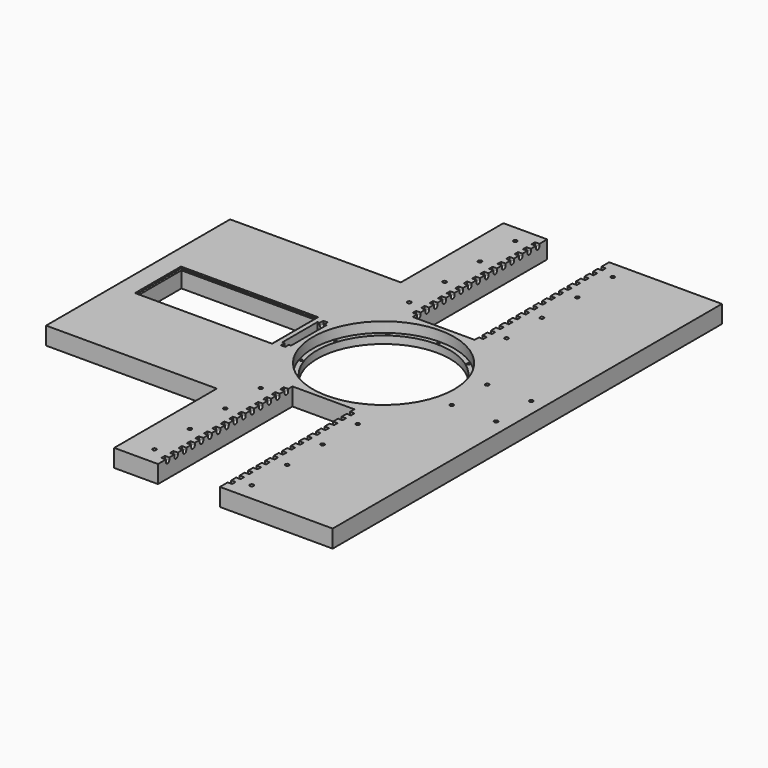
from build123d import *

# Parameters (mm, degrees)
F0_W      = 200
F0_H      = 255
F1_DEPTH  = 20
F2_W      = 150
F2_H      = 60
F3_DEPTH  = 20.001
F4_W      = 155
F4_H      = 65
F4_W_2    = 150
F4_H_2    = 60
F5_DEPTH  = 2
F6_DEPTH  = 240
F7_R      = 75
F8_DEPTH  = 25
F7_R_2    = 80
F9_DEPTH  = 11.5
F10_W     = 170
F10_H     = 147.5
F10_H_2   = 255
F10_R     = 80
F11_DEPTH = 10
F12_W     = 70
F12_H     = 190
F13_DEPTH = 25
F15_W     = 70
F15_H     = 190
F16_DEPTH = 25
F14_W     = 80
F14_H     = 5
F14_W_2   = 70
F14_H_2   = 6
F14_W_3   = 5
F14_H_3   = 7
F14_H_4   = 26.7300889492
F17_DEPTH = 5
F18_R     = 2.49999
F19_DEPTH = 147.5
F20_DEPTH = 147.5
F21_W     = 193
F21_H     = 20
F22_DEPTH = 145
F23_W     = 193
F23_H     = 20
F24_DEPTH = 145
F26_D     = 4.2
F26_DEPTH = 9.679
F26_TIP   = 1.2618073
F27_W     = 5
F27_H     = 60
F28_DEPTH = 5
F29_W     = 2.5
F29_H     = 50
F29_W_2   = 5
F30_DEPTH = 12
F31_R     = 2.49999
F33_D     = 4.2
F33_DEPTH = 9.679
F33_TIP   = 1.2618073
F34_R     = 75
F34_R_2   = 1.5
F35_DEPTH = 3


# Not quite as in the source:
# - a fillet or chamfer is up to 0.001 mm smaller than in the source, because OpenCascade refuses the exact size


with BuildPart() as f1:
    # F0 (on Top) → F1 (new body)
    with BuildSketch(Plane.XY):
        Rectangle(F0_W, F0_H)
    extrude(amount=F1_DEPTH)

    # F2 (on face) → F3 (cut, through all)
    with BuildSketch(Plane.XY.offset(20)):
        Rectangle(F2_W, F2_H)
    extrude(amount=-F3_DEPTH, mode=Mode.SUBTRACT)

    # F4 (on face) → F5 (cut)
    with BuildSketch(Plane.XY.offset(20)):
        Rectangle(F4_W, F4_H)
        Rectangle(F4_W_2, F4_H_2, mode=Mode.SUBTRACT)
    extrude(amount=-F5_DEPTH, mode=Mode.SUBTRACT)

    # F6 (add): a face of the model
    f6_faces = [f1.faces().sort_by_distance(p)[0] for p in [
        (100, 0, 10),
    ]]
    extrude(f6_faces, amount=F6_DEPTH)

    # F7 (on face) → F8 (cut)
    with BuildSketch(Plane.XY.offset(20)):
        with Locations((177.5, 0)):
            Circle(F7_R)
    extrude(amount=-F8_DEPTH, mode=Mode.SUBTRACT)

    # F7 (on face) → F9 (cut)
    with BuildSketch(Plane.XY.offset(20)):
        with Locations((177.5, 0)):
            Circle(F7_R_2)
        with Locations((177.5, 0)):
            Circle(F7_R, mode=Mode.SUBTRACT)
    extrude(amount=-F9_DEPTH, mode=Mode.SUBTRACT)

    # F10 (on face) → F11 (join)
    with BuildSketch(Plane.XY.offset(20)):
        with Locations((177.5, -201.25)):
            Rectangle(F10_W, F10_H)
        with Locations((177.5, 201.25)):
            Rectangle(F10_W, F10_H)
        with Locations((177.5, 0)):
            Rectangle(F10_W, F10_H_2)
        with Locations((177.5, 0)):
            Circle(F10_R, mode=Mode.SUBTRACT)
    extrude(amount=-F11_DEPTH)

    # F12 (on face) → F13 (cut)
    with BuildSketch(Plane.XY.offset(20)):
        with Locations((177.5, 180)):
            Rectangle(F12_W, F12_H)
    extrude(amount=-F13_DEPTH, mode=Mode.SUBTRACT)

    # F15 (on face) → F16 (cut)
    with BuildSketch(Plane.XY.offset(20)):
        with Locations((177.5, -180)):
            Rectangle(F15_W, F15_H)
    extrude(amount=-F16_DEPTH, mode=Mode.SUBTRACT)

    # F14 (on face) → F17 (cut)
    with BuildSketch(Plane.XY.offset(20)):
        with Locations((177.5, 93.5)):
            Rectangle(F14_W, F14_H)
        with Locations((177.5, 105.5)):
            Rectangle(F14_W, F14_H)
        with Locations((177.5, 117.5)):
            Rectangle(F14_W, F14_H)
        with Locations((177.5, 129.5)):
            Rectangle(F14_W, F14_H)
        with Locations((177.5, 141.5)):
            Rectangle(F14_W, F14_H)
        with Locations((177.5, 153.5)):
            Rectangle(F14_W, F14_H)
        with Locations((177.5, 165.5)):
            Rectangle(F14_W, F14_H)
        with Locations((177.5, 177.5)):
            Rectangle(F14_W, F14_H)
        with Locations((177.5, 189.5)):
            Rectangle(F14_W, F14_H)
        with Locations((177.5, 201.5)):
            Rectangle(F14_W, F14_H)
        with Locations((177.5, 213.5)):
            Rectangle(F14_W, F14_H)
        with Locations((177.5, 225.5)):
            Rectangle(F14_W, F14_H)
        with Locations((177.5, 237.5)):
            Rectangle(F14_W, F14_H)
        with Locations((177.5, 249.5)):
            Rectangle(F14_W, F14_H)
        with Locations((177.5, 261.5)):
            Rectangle(F14_W, F14_H)
        with Locations((177.5, -88)):
            Rectangle(F14_W_2, F14_H_2)
        with Locations((177.5, -93.5)):
            Rectangle(F14_W_2, F14_H)
        with Locations((140, -93.5)):
            Rectangle(F14_W_3, F14_H)
        with Locations((215, -93.5)):
            Rectangle(F14_W_3, F14_H)
        with Locations((177.5, -99.5)):
            Rectangle(F14_W_2, F14_H_3)
        with Locations((177.5, -105.5)):
            Rectangle(F14_W_2, F14_H)
        with Locations((140, -105.5)):
            Rectangle(F14_W_3, F14_H)
        with Locations((215, -105.5)):
            Rectangle(F14_W_3, F14_H)
        with Locations((177.5, -111.5)):
            Rectangle(F14_W_2, F14_H_3)
        with Locations((177.5, -117.5)):
            Rectangle(F14_W_2, F14_H)
        with Locations((140, -117.5)):
            Rectangle(F14_W_3, F14_H)
        with Locations((215, -117.5)):
            Rectangle(F14_W_3, F14_H)
        with Locations((177.5, -123.5)):
            Rectangle(F14_W_2, F14_H_3)
        with Locations((177.5, -129.5)):
            Rectangle(F14_W_2, F14_H)
        with Locations((140, -129.5)):
            Rectangle(F14_W_3, F14_H)
        with Locations((215, -129.5)):
            Rectangle(F14_W_3, F14_H)
        with Locations((177.5, -135.5)):
            Rectangle(F14_W_2, F14_H_3)
        with Locations((177.5, -141.5)):
            Rectangle(F14_W_2, F14_H)
        with Locations((140, -141.5)):
            Rectangle(F14_W_3, F14_H)
        with Locations((215, -141.5)):
            Rectangle(F14_W_3, F14_H)
        with Locations((177.5, -147.5)):
            Rectangle(F14_W_2, F14_H_3)
        with Locations((177.5, -153.5)):
            Rectangle(F14_W_2, F14_H)
        with Locations((140, -153.5)):
            Rectangle(F14_W_3, F14_H)
        with Locations((215, -153.5)):
            Rectangle(F14_W_3, F14_H)
        with Locations((177.5, -159.5)):
            Rectangle(F14_W_2, F14_H_3)
        with Locations((177.5, -165.5)):
            Rectangle(F14_W_2, F14_H)
        with Locations((140, -165.5)):
            Rectangle(F14_W_3, F14_H)
        with Locations((215, -165.5)):
            Rectangle(F14_W_3, F14_H)
        with Locations((177.5, -171.5)):
            Rectangle(F14_W_2, F14_H_3)
        with Locations((177.5, -177.5)):
            Rectangle(F14_W_2, F14_H)
        with Locations((140, -177.5)):
            Rectangle(F14_W_3, F14_H)
        with Locations((215, -177.5)):
            Rectangle(F14_W_3, F14_H)
        with Locations((177.5, -183.5)):
            Rectangle(F14_W_2, F14_H_3)
        with Locations((177.5, -189.5)):
            Rectangle(F14_W_2, F14_H)
        with Locations((140, -189.5)):
            Rectangle(F14_W_3, F14_H)
        with Locations((215, -189.5)):
            Rectangle(F14_W_3, F14_H)
        with Locations((177.5, -195.5)):
            Rectangle(F14_W_2, F14_H_3)
        with Locations((177.5, -201.5)):
            Rectangle(F14_W_2, F14_H)
        with Locations((140, -201.5)):
            Rectangle(F14_W_3, F14_H)
        with Locations((215, -201.5)):
            Rectangle(F14_W_3, F14_H)
        with Locations((177.5, -207.5)):
            Rectangle(F14_W_2, F14_H_3)
        with Locations((177.5, -213.5)):
            Rectangle(F14_W_2, F14_H)
        with Locations((140, -213.5)):
            Rectangle(F14_W_3, F14_H)
        with Locations((215, -213.5)):
            Rectangle(F14_W_3, F14_H)
        with Locations((177.5, -219.5)):
            Rectangle(F14_W_2, F14_H_3)
        with Locations((177.5, -225.5)):
            Rectangle(F14_W_2, F14_H)
        with Locations((140, -225.5)):
            Rectangle(F14_W_3, F14_H)
        with Locations((215, -225.5)):
            Rectangle(F14_W_3, F14_H)
        with Locations((177.5, -231.5)):
            Rectangle(F14_W_2, F14_H_3)
        with Locations((177.5, -237.5)):
            Rectangle(F14_W_2, F14_H)
        with Locations((140, -237.5)):
            Rectangle(F14_W_3, F14_H)
        with Locations((215, -237.5)):
            Rectangle(F14_W_3, F14_H)
        with Locations((177.5, -243.5)):
            Rectangle(F14_W_2, F14_H_3)
        with Locations((177.5, -249.5)):
            Rectangle(F14_W_2, F14_H)
        with Locations((140, -249.5)):
            Rectangle(F14_W_3, F14_H)
        with Locations((215, -249.5)):
            Rectangle(F14_W_3, F14_H)
        with Locations((177.5, -255.5)):
            Rectangle(F14_W_2, F14_H_3)
        with Locations((177.5, -261.5)):
            Rectangle(F14_W_2, F14_H)
        with Locations((140, -261.5)):
            Rectangle(F14_W_3, F14_H)
        with Locations((215, -261.5)):
            Rectangle(F14_W_3, F14_H)
        with Locations((177.5, -277.3650444746)):
            Rectangle(F14_W_2, F14_H_4)
    extrude(amount=-F17_DEPTH, mode=Mode.SUBTRACT)

    # F18 (radius 2.5 in the source; OpenCascade refuses exactly that, so slightly less here)
    f18_edges = [f1.edges().sort_by_distance(p)[0] for p in [
        (140, 264, 15),
        (140, 259, 15),
        (140, 252, 15),
        (140, 247, 15),
        (140, 235, 15),
        (140, 240, 15),
        (140, 228, 15),
        (140, 223, 15),
        (140, 211, 15),
        (140, 216, 15),
        (140, 204, 15),
        (140, 199, 15),
        (140, 192, 15),
        (140, 187, 15),
        (140, 180, 15),
        (140, 175, 15),
        (140, 168, 15),
        (140, 163, 15),
        (140, 156, 15),
        (140, 151, 15),
        (140, 144, 15),
        (140, 139, 15),
        (140, 132, 15),
        (140, 127, 15),
        (140, 120, 15),
        (140, 115, 15),
        (140, 108, 15),
        (140, 103, 15),
        (140, 96, 15),
        (140, 91, 15),
        (215, 96, 15),
        (215, 91, 15),
        (215, 108, 15),
        (215, 103, 15),
        (215, 120, 15),
        (215, 115, 15),
        (215, 132, 15),
        (215, 127, 15),
        (215, 144, 15),
        (215, 139, 15),
        (215, 156, 15),
        (215, 151, 15),
        (215, 168, 15),
        (215, 163, 15),
        (215, 180, 15),
        (215, 175, 15),
        (215, 192, 15),
        (215, 187, 15),
        (215, 204, 15),
        (215, 199, 15),
        (215, 216, 15),
        (215, 211, 15),
        (215, 228, 15),
        (215, 223, 15),
        (215, 240, 15),
        (215, 235, 15),
        (215, 252, 15),
        (215, 247, 15),
        (215, 264, 15),
        (215, 259, 15),
        (215, -264, 15),
        (215, -259, 15),
        (215, -247, 15),
        (215, -252, 15),
        (215, -235, 15),
        (215, -240, 15),
        (215, -223, 15),
        (215, -228, 15),
        (215, -211, 15),
        (215, -216, 15),
        (215, -199, 15),
        (215, -204, 15),
        (215, -187, 15),
        (215, -192, 15),
        (215, -175, 15),
        (215, -180, 15),
        (215, -163, 15),
        (215, -168, 15),
        (215, -151, 15),
        (215, -156, 15),
        (215, -139, 15),
        (215, -144, 15),
        (215, -127, 15),
        (215, -132, 15),
        (215, -115, 15),
        (215, -120, 15),
        (215, -103, 15),
        (215, -108, 15),
        (215, -91, 15),
        (215, -96, 15),
        (140, -259, 15),
        (140, -264, 15),
        (140, -252, 15),
        (140, -247, 15),
        (140, -240, 15),
        (140, -235, 15),
        (140, -223, 15),
        (140, -228, 15),
        (140, -211, 15),
        (140, -216, 15),
        (140, -199, 15),
        (140, -204, 15),
        (140, -192, 15),
        (140, -187, 15),
        (140, -163, 15),
        (140, -168, 15),
        (140, -175, 15),
        (140, -180, 15),
        (140, -156, 15),
        (140, -151, 15),
        (140, -139, 15),
        (140, -144, 15),
        (140, -127, 15),
        (140, -132, 15),
        (140, -115, 15),
        (140, -120, 15),
        (140, -103, 15),
        (140, -108, 15),
        (140, -91, 15),
    ]]
    fillet(f18_edges, radius=F18_R)

    # F19 (add): faces of the model
    f19_faces = [f1.faces().sort_by_distance(p)[0] for p in [
        (10.1867816092, -127.5, 9.4252873563),
        (285.7012195122, -127.5, 8.7804878049),
    ]]
    extrude(f19_faces, amount=F19_DEPTH)

    # F20 (add): faces of the model
    f20_faces = [f1.faces().sort_by_distance(p)[0] for p in [
        (10.1867816092, 127.5, 9.4252873563),
        (285.7012195122, 127.5, 8.7804878049),
    ]]
    extrude(f20_faces, amount=F20_DEPTH)

    # F21 (on face) → F22 (cut)
    with BuildSketch(Plane.XZ.offset(275)):
        with Locations((-3.5, 10)):
            Rectangle(F21_W, F21_H)
    extrude(amount=-F22_DEPTH, mode=Mode.SUBTRACT)

    # F23 (on face) → F24 (cut)
    with BuildSketch(Plane(origin=(0, 275, 0), x_dir=(-1, 0, 0), z_dir=(0, 1, 0))):
        with Locations((3.5, 10)):
            Rectangle(F23_W, F23_H)
    extrude(amount=-F24_DEPTH, mode=Mode.SUBTRACT)

    # F26
    with Locations(Plane.XY.offset(20)):
        with Locations((122.5, 105), (232.5, 105), (232.5, 155), (122.5, 155), (122.5, 205), (232.5, 205), (232.5, 255), (122.5, 255), (122.5, -255), (232.5, -255), (232.5, -205), (122.5, -205), (122.5, -155), (232.5, -155), (232.5, -105), (122.5, -105)):
            Hole(F26_D / 2, depth=F26_DEPTH)
            with Locations((0, 0, -(F26_DEPTH + F26_TIP / 2))):  # 118° drill point
                Cone(0, F26_D / 2, F26_TIP, mode=Mode.SUBTRACT)

    # F27 (on face) → F28 (cut)
    with BuildSketch(Plane.XY.offset(20)):
        with Locations((87.8393128514, 0)):
            Rectangle(F27_W, F27_H)
    extrude(amount=-F28_DEPTH, mode=Mode.SUBTRACT)

    # F29 (on face) → F30 (cut)
    with BuildSketch(Plane.XY.offset(20)):
        with Locations((91.5893128514, 0)):
            Rectangle(F29_W, F29_H)
        with Locations((84.0893128514, 0)):
            Rectangle(F29_W, F29_H)
        with Locations((87.8393128514, 0)):
            Rectangle(F29_W_2, F29_H)
    extrude(amount=-F30_DEPTH, mode=Mode.SUBTRACT)

    # F31 (radius 2.5 in the source; OpenCascade refuses exactly that, so slightly less here)
    f31_edges = [f1.edges().sort_by_distance(p)[0] for p in [
        (90.339313, 27.5, 15),
        (85.339313, 27.5, 15),
        (90.339313, -27.5, 15),
        (85.339313, -27.5, 15),
        (140, -96, 15),
    ]]
    fillet(f31_edges, radius=F31_R)

    # F33
    with Locations(Plane.XY.offset(20)):
        with Locations((274.6371090412, 25), (324.6371090412, 25), (324.6371090412, -25), (274.6371090412, -25)):
            Hole(F33_D / 2, depth=F33_DEPTH)
            with Locations((0, 0, -(F33_DEPTH + F33_TIP / 2))):  # 118° drill point
                Cone(0, F33_D / 2, F33_TIP, mode=Mode.SUBTRACT)

    # F34 (on face) → F35 (cut)
    with BuildSketch(Plane.XY.offset(8.5)):
        with Locations((177.5, 0)):
            Circle(F34_R)
        with Locations((177.5, 77.5)):
            Circle(F34_R_2)
        with Locations((131.9466429473, 62.6988170641)):
            Circle(F34_R_2)
        with Locations((103.7931199871, 23.9488170641)):
            Circle(F34_R_2)
        with Locations((103.7931199871, -23.9488170641)):
            Circle(F34_R_2)
        with Locations((131.9466429473, -62.6988170641)):
            Circle(F34_R_2)
        with Locations((177.5, -77.5)):
            Circle(F34_R_2)
        with Locations((223.0533570527, -62.6988170641)):
            Circle(F34_R_2)
        with Locations((251.2068800129, -23.9488170641)):
            Circle(F34_R_2)
        with Locations((251.2068800129, 23.9488170641)):
            Circle(F34_R_2)
        with Locations((223.0533570527, 62.6988170641)):
            Circle(F34_R_2)
    extrude(amount=-F35_DEPTH, mode=Mode.SUBTRACT)


solid = f1.part
